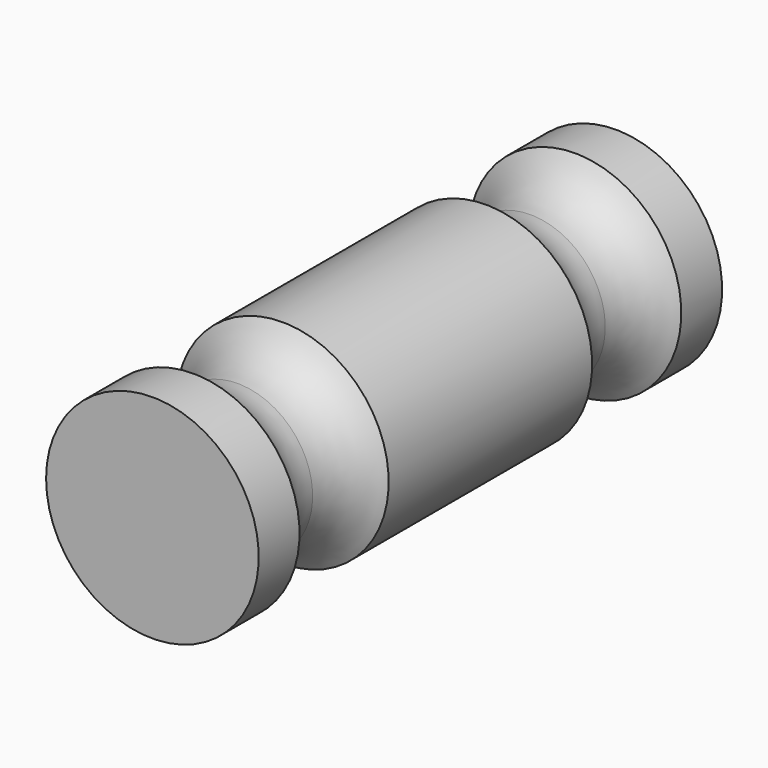
from build123d import *

# Parameters (mm, degrees)
F0_W   = 2.2352
F0_H   = 1.524
F0_W_2 = 0.9398
F0_H_2 = 7.5946


# Not quite as in the source:
# - a feature names something its author has since deleted; it is built from what else it names


with BuildPart() as f1:
    # F0 (on Top) → F1 (revolve)
    with BuildSketch(Plane.XY):
        with Locations((1.1176, 7.8867)):
            Rectangle(F0_W, F0_H)
        Polygon((2.2352, 7.1247), (0, 7.1247), (0, 3.7973), (2.2352, 3.7973), (2.2352, 5.4609999998), align=None)
        with Locations((-2.7051, 7.8867)):
            Rectangle(F0_W_2, F0_H)
        with Locations((1.1176, 0)):
            Rectangle(F0_W, F0_H_2)
        with BuildLine():
            Line((-2.2352, 5.461), (-2.2352, 7.1247))
            Line((-2.2352, 7.1247), (-3.175, 7.1247))
            ThreePointArc((-3.175, 7.1247), (-2.4863911938, 6.4163954325), (-2.2352, 5.461))
        make_face()
        Polygon((2.2352, -3.7973), (0, -3.7973), (0, -7.1247), (2.2352, -7.1247), (2.2352, -5.4610000002), align=None)
        with BuildLine():
            Line((-3.175, 3.7973), (-2.2352, 3.7973))
            Line((-2.2352, 3.7973), (-2.2352, 5.461))
            ThreePointArc((-2.2352, 5.461), (-2.4863911938, 4.5056045675), (-3.175, 3.7973))
        make_face()
        with Locations((-2.7051, 0)):
            Rectangle(F0_W_2, F0_H_2)
        with Locations((1.1176, -7.8867)):
            Rectangle(F0_W, F0_H)
        with BuildLine():
            Line((-2.2352, -5.461), (-2.2352, -3.7973))
            Line((-2.2352, -3.7973), (-3.175, -3.7973))
            ThreePointArc((-3.175, -3.7973), (-2.4863911938, -4.5056045675), (-2.2352, -5.461))
        make_face()
        with Locations((-2.7051, -7.8867)):
            Rectangle(F0_W_2, F0_H)
        with BuildLine():
            Line((-3.175, -7.1247), (-2.2352, -7.1247))
            Line((-2.2352, -7.1247), (-2.2352, -5.461))
            ThreePointArc((-2.2352, -5.461), (-2.4863911938, -6.4163954325), (-3.175, -7.1247))
        make_face()
        with Locations((2.7051, -7.8867)):
            Rectangle(F0_W_2, F0_H)
    revolve(axis=Axis((0, 0, 0), (0, 1, 0)))


solid = f1.part
